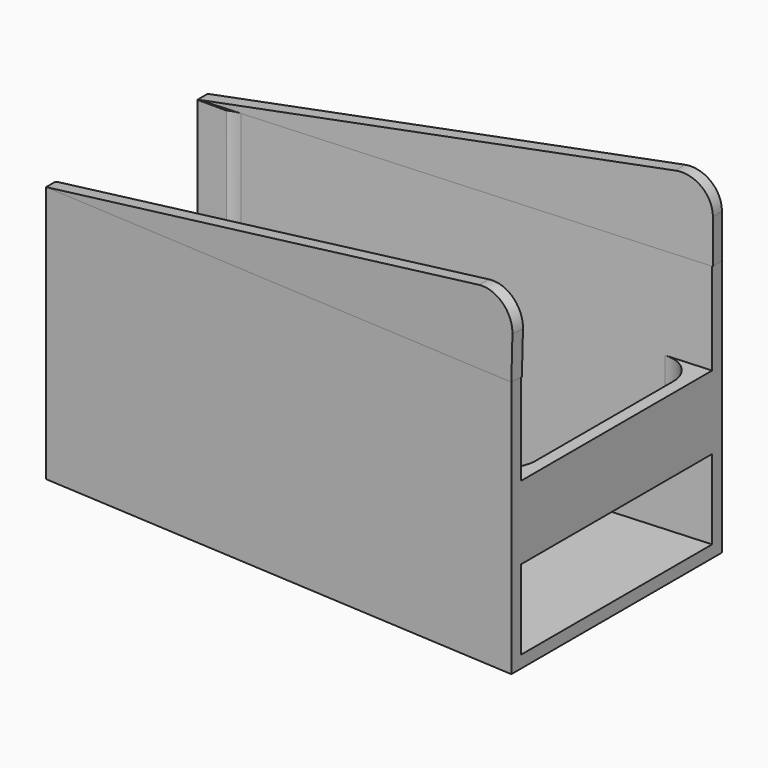
from build123d import *

# Parameters (mm, degrees)
F1_DEPTH      = 2
F2_DEPTH      = 42
F5_DEPTH      = 2
F7_DEPTH      = 2
F8_W          = 28.9586056024
F8_H          = 21
F9_DEPTH      = 25
F10_W         = 38.9921951145
F10_H         = 12
F11_DEPTH     = 2
F12_T1_DEPTH  = 12
F12_T6_DEPTH  = 51.7431402671
F12_T11_DEPTH = 51.7431402671
F12_T17_DEPTH = 40
F12_T22_DEPTH = 51.7431402671
F13_R         = 5


# Not quite as in the source:
# - a fillet or chamfer that OpenCascade refuses, or shapes differently, is made with other operations: its cross-section is extruded or revolved along the edge and cut away or added


with BuildPart() as f1:
    # F0 (on Top) → F1 (new body)
    with BuildSketch(Plane.XY):
        Polygon((16.9007111498, 56.5512960928), (-61.0992888502, 51.6762960928), (-61.0992888502, 18.6762960928), (16.9007111498, 13.8012960928), (18.9007111498, 13.6762960928), (18.9007111498, 15.6801985355), (16.9007111498, 15.8051985355), (-59.0992888502, 20.5551985355), (-59.0992888502, 49.79739365), (16.9007111498, 54.54739365), (18.9007111498, 54.67239365), (18.9007111498, 56.6762960928), align=None)
        Polygon((18.9007111498, 15.6801985355), (18.9007111498, 54.67239365), (16.9007111498, 54.54739365), (16.9007111498, 15.8051985355), align=None)
        Polygon((16.9007111498, 15.8051985355), (16.9007111498, 54.54739365), (-59.0992888502, 49.79739365), (-59.0992888502, 20.5551985355), align=None)
    extrude(amount=F1_DEPTH)

    # F0 (on Top) → F2 (join)
    with BuildSketch(Plane.XY):
        Polygon((16.9007111498, 56.5512960928), (-61.0992888502, 51.6762960928), (-61.0992888502, 18.6762960928), (16.9007111498, 13.8012960928), (18.9007111498, 13.6762960928), (18.9007111498, 15.6801985355), (16.9007111498, 15.8051985355), (-59.0992888502, 20.5551985355), (-59.0992888502, 49.79739365), (16.9007111498, 54.54739365), (18.9007111498, 54.67239365), (18.9007111498, 56.6762960928), align=None)
    extrude(amount=F2_DEPTH)

    # F3 (on face) → F5 (join)
    with BuildSketch(Plane(origin=(0.9249861815, 14.7997789033, 0), x_dir=(0.9980525785, -0.0623782862, 0), z_dir=(-0.0623782862, -0.9980525785, 0))):
        Polygon((18.3653086424, 55), (-62.1452981224, 42), (18.010799587, 42), align=None)
    extrude(amount=-F5_DEPTH)

    # F6 (on face) → F7 (join)
    with BuildSketch(Plane(origin=(-3.4549417367, 55.2790677874, 0), x_dir=(-0.9980525785, -0.0623782862, 0), z_dir=(-0.0623782862, 0.9980525785, 0))):
        Polygon((-22.3992737141, 55), (-22.3992737141, 42), (57.7568239953, 42), align=None)
    extrude(amount=-F7_DEPTH)

    # F8 (on face) → F9 (cut)
    with BuildSketch(Plane(origin=(-61.0992888502, 0, 0), x_dir=(0, -1, 0), z_dir=(-1, 0, 0))):
        with Locations((-35.0762708113, 31.5)):
            Rectangle(F8_W, F8_H)
    extrude(amount=-F9_DEPTH, mode=Mode.SUBTRACT)

    # F10 (on face) → F11 (join)
    with BuildSketch(Plane.YZ.offset(18.9007111498)):
        with Locations((35.1762960928, 21)):
            Rectangle(F10_W, F10_H)
    extrude(amount=-F11_DEPTH)

    # F12: fillet of radius 5 on 4 edges, made by hand

    # F12_s2 → F12_t1 (join)
    with BuildSketch(Plane.XY.offset(15)):
        with BuildLine():
            ThreePointArc((11.588819719, 16.1371917499), (15.324199345, 17.4833184516), (16.9007111498, 21.1274546423))
            Line((16.9007111498, 21.1274546423), (16.9007111498, 15.8051985355))
            Line((16.9007111498, 15.8051985355), (11.588819719, 16.1371917499))
        make_face()
        with BuildLine():
            ThreePointArc((11.588819719, 54.2154004356), (15.324199345, 52.869273734), (16.9007111498, 49.2251375432))
            Line((16.9007111498, 49.2251375432), (16.9007111498, 54.54739365))
            Line((16.9007111498, 54.54739365), (11.588819719, 54.2154004356))
        make_face()
    extrude(amount=F12_T1_DEPTH)


with BuildPart() as f12_tool4:
    # F12_s5 → F12_t6 (new body)
    with BuildSketch(Plane.XY.offset(2)):
        with BuildLine():
            ThreePointArc((-54.411180281, 20.2621917499), (-57.743425041, 21.8289664471), (-59.0992888502, 25.2524546423))
            Line((-59.0992888502, 25.2524546423), (-59.0992888502, 20.5551985355))
            Line((-59.0992888502, 20.5551985355), (-54.411180281, 20.2621917499))
        make_face()
    extrude(amount=F12_T6_DEPTH)

    split(bisect_by=Plane.XY.offset(21), keep=Keep.BOTTOM)


with BuildPart() as f1_1:
    add(f1.part)

    # F12_t3: union F12_tool4
    add(f12_tool4.part)


with BuildPart() as f12_tool9:
    # F12_s10 → F12_t11 (new body)
    with BuildSketch(Plane.XY.offset(-9.7431402671)):
        with BuildLine():
            ThreePointArc((-54.411180281, 20.2621917499), (-57.743425041, 21.8289664471), (-59.0992888502, 25.2524546423))
            Line((-59.0992888502, 25.2524546423), (-59.0992888502, 20.5551985355))
            Line((-59.0992888502, 20.5551985355), (-54.411180281, 20.2621917499))
        make_face()
    extrude(amount=F12_T11_DEPTH)

    split(bisect_by=Plane.XZ.offset(-20.5969680101), keep=Keep.TOP)

    split(bisect_by=Plane.XY.offset(21), keep=Keep.TOP)


with BuildPart() as f1_2:
    add(f1_1.part)

    # F12_t8: union F12_tool9
    add(f12_tool9.part)


with BuildPart() as f12_tool15:
    # F12_s16 → F12_t17 (new body)
    with BuildSketch(Plane.XY.offset(2)):
        with BuildLine():
            ThreePointArc((-54.411180281, 50.0904004356), (-57.743425041, 48.5236257384), (-59.0992888502, 45.1001375432))
            Line((-59.0992888502, 45.1001375432), (-59.0992888502, 49.79739365))
            Line((-59.0992888502, 49.79739365), (-54.411180281, 50.0904004356))
        make_face()
    extrude(amount=F12_T17_DEPTH)

    split(bisect_by=Plane.XZ.offset(-49.5555736125), keep=Keep.BOTTOM)


with BuildPart() as f1_3:
    add(f1_2.part)

    # F12_t14: union F12_tool15
    add(f12_tool15.part)


with BuildPart() as f12_tool20:
    # F12_s21 → F12_t22 (new body)
    with BuildSketch(Plane.XY.offset(2)):
        with BuildLine():
            ThreePointArc((-54.411180281, 50.0904004356), (-57.743425041, 48.5236257384), (-59.0992888502, 45.1001375432))
            Line((-59.0992888502, 45.1001375432), (-59.0992888502, 49.79739365))
            Line((-59.0992888502, 49.79739365), (-54.411180281, 50.0904004356))
        make_face()
    extrude(amount=F12_T22_DEPTH)

    split(bisect_by=Plane.XY.offset(21), keep=Keep.BOTTOM)


with BuildPart() as f1_4:
    add(f1_3.part)

    # F12_t19: union F12_tool20
    add(f12_tool20.part)

    # F13
    f13_edges = [f1_4.edges().sort_by_distance(p)[0] for p in [
        (18.963089, 55.678244, 55),
        (19.316908, 14.652235, 55),
    ]]
    fillet(f13_edges, radius=F13_R)


solid = f1_4.part
